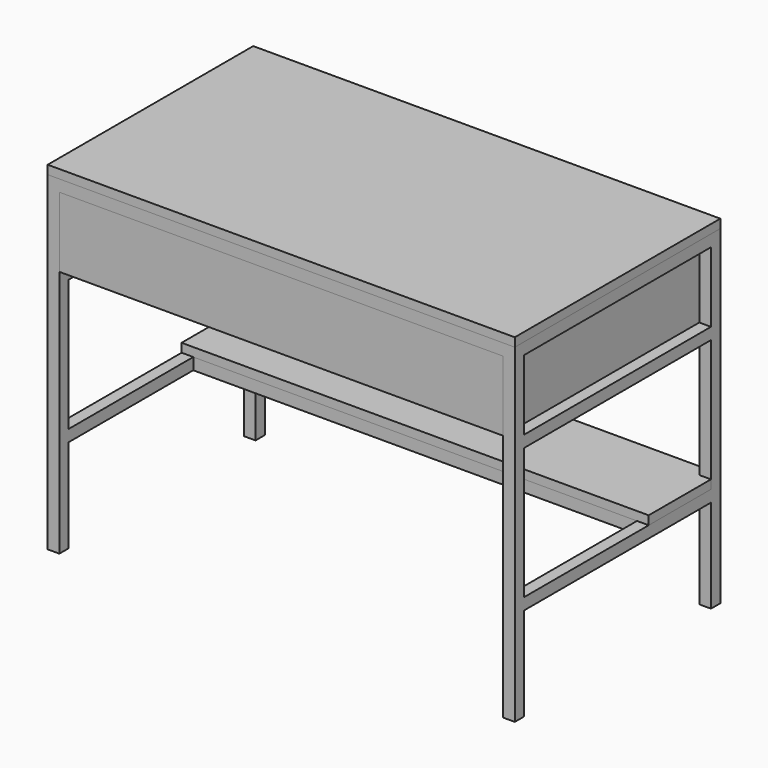
from build123d import *

# Parameters (mm, degrees)
F4_W      = 1016
F4_H      = 558.8
F4_W_2    = 25.4
F4_H_2    = 508
F5_DEPTH  = 25.4
F6_W      = 1016
F6_H      = 558.8
F7_DEPTH  = 19.05
F8_W      = 25.4
F8_H      = 25.4
F9_DEPTH  = 692.15
F10_W     = 25.4
F10_H     = 25.4
F11_DEPTH = 508
F12_W     = 25.4
F12_H     = 25.4
F13_DEPTH = 508
F14_W     = 25.4
F14_H     = 25.4
F15_DEPTH = 965.2
F16_W     = 25.4
F16_H     = 25.4
F17_DEPTH = 143.9333333333
F19_DEPTH = 19.05
F20_W     = 25.4
F20_H     = 25.4
F21_DEPTH = 508
F22_W     = 25.4
F22_H     = 25.4
F23_DEPTH = 508
F24_W     = 508
F24_H     = 152.4
F24_W_2   = 25.4
F25_DEPTH = 965.2


# Not quite as in the source:
# - a length typed as a fraction of an inch, garbled in the dataset ("3 / 203.2 mm" for 3/8 in), is restored


with BuildPart() as f5:
    # F4 (on Top) → F5 (new body)
    with BuildSketch(Plane.XY):
        Rectangle(F4_W, F4_H)
        Polygon((482.6, 254), (482.6, -254), (186.2666666667, -254), (160.8666666667, -254), (-148.1666666667, -254), (-173.5666666667, -254), (-482.6, -254), (-482.6, 254), (-173.5666666667, 254), (-148.1666666667, 254), (160.8666666667, 254), (186.2666666667, 254), align=None, mode=Mode.SUBTRACT)
        with Locations((-160.8666666667, 0)):
            Rectangle(F4_W_2, F4_H_2)
        with Locations((173.5666666667, 0)):
            Rectangle(F4_W_2, F4_H_2)
    extrude(amount=F5_DEPTH)

    # F8 (on face) → F9 (join)
    with BuildSketch(Plane(origin=(0, 0, 0), x_dir=(1, 0, 0), z_dir=(0, 0, -1))):
        with Locations((-495.3, 266.7)):
            Rectangle(F8_W, F8_H)
        with Locations((-495.3, -266.7)):
            Rectangle(F8_W, F8_H)
        with Locations((495.3, 266.7)):
            Rectangle(F8_W, F8_H)
        with Locations((495.3, -266.7)):
            Rectangle(F8_W, F8_H)
    extrude(amount=F9_DEPTH)

    # F10 (on face) → F11 (join, through all)
    with BuildSketch(Plane.XZ.offset(-254)):
        with Locations((-495.3, -476.25)):
            Rectangle(F10_W, F10_H)
    extrude(amount=F11_DEPTH)

    # F12 (on face) → F13 (join, through all)
    with BuildSketch(Plane.XZ.offset(-254)):
        with Locations((495.3, -476.25)):
            Rectangle(F12_W, F12_H)
    extrude(amount=F13_DEPTH)

    # F14 (on face) → F15 (join, through all)
    with BuildSketch(Plane(origin=(482.6, 0, 0), x_dir=(0, -1, 0), z_dir=(-1, 0, 0))):
        with Locations((-97.3666666667, -476.25)):
            Rectangle(F14_W, F14_H)
        with Locations((-266.7, -476.25)):
            Rectangle(F14_W, F14_H)
    extrude(amount=F15_DEPTH)

    # F16 (on face) → F17 (join, through all)
    with BuildSketch(Plane.XZ.offset(-254)):
        with Locations((-160.8666666667, -476.25)):
            Rectangle(F16_W, F16_H)
        with Locations((173.5666666667, -476.25)):
            Rectangle(F16_W, F16_H)
    extrude(amount=F17_DEPTH)

    # F20 (on face) → F21 (join, through all)
    with BuildSketch(Plane.XZ.offset(-254)):
        with Locations((-495.3, -165.1)):
            Rectangle(F20_W, F20_H)
    extrude(amount=F21_DEPTH)

    # F22 (on face) → F23 (join, through all)
    with BuildSketch(Plane.XZ.offset(-254)):
        with Locations((495.3, -165.1)):
            Rectangle(F22_W, F22_H)
    extrude(amount=F23_DEPTH)


with BuildPart() as f7:
    # F6 (on face) → F7 (new body)
    with BuildSketch(Plane.XY.offset(25.4)):
        Rectangle(F6_W, F6_H)
    extrude(amount=F7_DEPTH)


with BuildPart() as f19:
    # F18 (on face) → F19 (new body)
    with BuildSketch(Plane.XY.offset(-463.55)):
        Polygon((-482.6, 254), (-508, 254), (-508, 84.6666666667), (508, 84.6666666667), (508, 254), (482.6, 254), (482.6, 279.4), (-482.6, 279.4), align=None)
    extrude(amount=F19_DEPTH)


with BuildPart() as f25:
    # F24 (on face) → F25 (new body)
    with BuildSketch(Plane.YZ.offset(-482.6)):
        with Locations((0, -76.2)):
            Rectangle(F24_W, F24_H)
        with Locations((-266.7, -76.2)):
            Rectangle(F24_W_2, F24_H)
    extrude(amount=F25_DEPTH)


solid = Compound([f5.part, f7.part, f19.part, f25.part])
